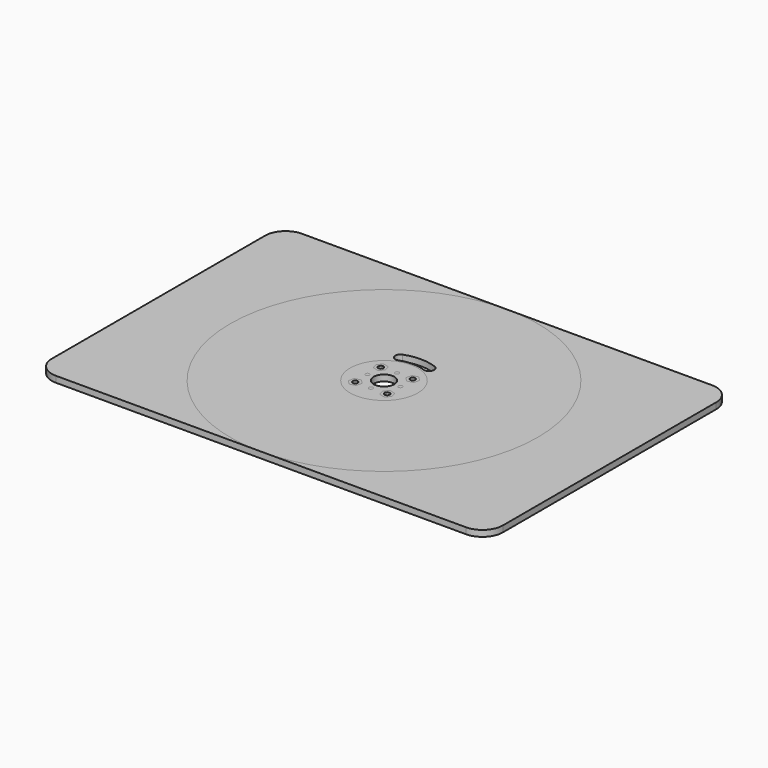
from build123d import *

# Parameters (mm, degrees)
F12_DEPTH = 3
F2_W      = 29
F2_H      = 59.5
F2_R      = 1.25
F6_R      = 2
F13_DEPTH = 25
F3_R      = 75
F14_DEPTH = 3
F5_R      = 2
F7_R      = 30
F15_DEPTH = 25
F16_DEPTH = 3
F0_R      = 5
F0_R_2    = 1.25
F17_DEPTH = 25
F9_R      = 16.5
F18_DEPTH = 3
F11_R     = 1
F19_DEPTH = 25
F20_DEPTH = 3
F10_R     = 2
F21_DEPTH = 25
F22_DEPTH = 3
F1_R      = 5
F23_DEPTH = 25


with BuildPart() as f12:
    # F4 (on Top) → F12 (new body)
    with BuildSketch(Plane.XY):
        with BuildLine():
            Line((100, 75), (-100, 75))
            ThreePointArc((-100, 75), (-107.0710678119, 72.0710678119), (-110, 65))
            Line((-110, 65), (-110, -65))
            ThreePointArc((-110, -65), (-107.0710678119, -72.0710678119), (-100, -75))
            Line((-100, -75), (100, -75))
            ThreePointArc((100, -75), (107.0710678119, -72.0710678119), (110, -65))
            Line((110, -65), (110, 65))
            ThreePointArc((110, 65), (107.0710678119, 72.0710678119), (100, 75))
        make_face()
    extrude(amount=F12_DEPTH)

    # F2 (on Top) + F6 (on Top) + F8 (on Top) → F13 (cut)
    with BuildSketch(Plane.XY):
        with Locations((0, -15.25)):
            Rectangle(F2_W, F2_H)
        with Locations((17.3, 4)):
            Circle(F2_R)
        with Locations((17.3, -18)):
            Circle(F2_R)
        with Locations((17.3, -40)):
            Circle(F2_R)
        with Locations((-17.3, 4)):
            Circle(F2_R)
        with Locations((-17.3, -18)):
            Circle(F2_R)
        with Locations((-17.3, -40)):
            Circle(F2_R)
        with Locations((11, -47.8)):
            Circle(F2_R)
        with Locations((-11, -47.8)):
            Circle(F2_R)
    with BuildSketch(Plane.XY):
        with Locations((38.1837661841, 38.1837661841)):
            Circle(F6_R)
        with Locations((-38.1837661841, 38.1837661841)):
            Circle(F6_R)
        with Locations((-38.1837661841, -38.1837661841)):
            Circle(F6_R)
        with Locations((38.1837661841, -38.1837661841)):
            Circle(F6_R)
    with BuildSketch(Plane.XY):
        with BuildLine():
            ThreePointArc((-7.875, 21.0768682446), (-9.3418742494, 17.8599939952), (-6.125, 16.3931197458))
            ThreePointArc((-6.125, 16.3931197458), (0, 17.5), (6.125, 16.3931197458))
            ThreePointArc((6.125, 16.3931197458), (9.3418742494, 17.8599939952), (7.875, 21.0768682446))
            ThreePointArc((7.875, 21.0768682446), (0, 22.5), (-7.875, 21.0768682446))
        make_face()
    extrude(amount=F13_DEPTH, mode=Mode.SUBTRACT)


with BuildPart() as f14:
    # F3 (on Top) → F14 (new body)
    with BuildSketch(Plane.XY):
        Circle(F3_R)
    extrude(amount=F14_DEPTH)

    # F5 (on Top) + F7 (on Top) → F15 (cut)
    with BuildSketch(Plane.XY):
        with Locations((0, 54)):
            Circle(F5_R)
        with Locations((-54, 0)):
            Circle(F5_R)
        with Locations((0, -54)):
            Circle(F5_R)
        with Locations((54, 0)):
            Circle(F5_R)
    with BuildSketch(Plane.XY):
        Circle(F7_R)
    extrude(amount=F15_DEPTH, mode=Mode.SUBTRACT)


with BuildPart() as f16:
    # F3 (on Top) → F16 (new body)
    with BuildSketch(Plane.XY):
        Circle(F3_R)
    extrude(amount=F16_DEPTH)

    # F0 (on Top) + F8 (on Top) → F17 (cut)
    with BuildSketch(Plane.XY):
        Circle(F0_R)
        with Locations((7.7781745931, 7.7781745931)):
            Circle(F0_R_2)
        with Locations((-7.7781745931, 7.7781745931)):
            Circle(F0_R_2)
        with Locations((-7.7781745931, -7.7781745931)):
            Circle(F0_R_2)
        with Locations((7.7781745931, -7.7781745931)):
            Circle(F0_R_2)
    with BuildSketch(Plane.XY):
        with BuildLine():
            ThreePointArc((-7.875, 21.0768682446), (-9.3418742494, 17.8599939952), (-6.125, 16.3931197458))
            ThreePointArc((-6.125, 16.3931197458), (0, 17.5), (6.125, 16.3931197458))
            ThreePointArc((6.125, 16.3931197458), (9.3418742494, 17.8599939952), (7.875, 21.0768682446))
            ThreePointArc((7.875, 21.0768682446), (0, 22.5), (-7.875, 21.0768682446))
        make_face()
    extrude(amount=F17_DEPTH, mode=Mode.SUBTRACT)


with BuildPart() as f18:
    # F9 (on Top) → F18 (new body)
    with BuildSketch(Plane.XY):
        Circle(F9_R)
    extrude(amount=F18_DEPTH)

    # F0 (on Top) + F11 (on Top) → F19 (cut)
    with BuildSketch(Plane.XY):
        Circle(F0_R)
        with Locations((7.7781745931, 7.7781745931)):
            Circle(F0_R_2)
        with Locations((-7.7781745931, 7.7781745931)):
            Circle(F0_R_2)
        with Locations((-7.7781745931, -7.7781745931)):
            Circle(F0_R_2)
        with Locations((7.7781745931, -7.7781745931)):
            Circle(F0_R_2)
    with BuildSketch(Plane.XY):
        with Locations((0, 8)):
            Circle(F11_R)
        with Locations((-8, 0)):
            Circle(F11_R)
        with Locations((0, -8)):
            Circle(F11_R)
        with Locations((8, 0)):
            Circle(F11_R)
    extrude(amount=F19_DEPTH, mode=Mode.SUBTRACT)


with BuildPart() as f20:
    # F9 (on Top) → F20 (new body)
    with BuildSketch(Plane.XY):
        Circle(F9_R)
    extrude(amount=F20_DEPTH)

    # F0 (on Top) + F10 (on Top) → F21 (cut)
    with BuildSketch(Plane.XY):
        Circle(F0_R)
        with Locations((7.7781745931, 7.7781745931)):
            Circle(F0_R_2)
        with Locations((-7.7781745931, 7.7781745931)):
            Circle(F0_R_2)
        with Locations((-7.7781745931, -7.7781745931)):
            Circle(F0_R_2)
        with Locations((7.7781745931, -7.7781745931)):
            Circle(F0_R_2)
    with BuildSketch(Plane.XY):
        with Locations((0, 8)):
            Circle(F10_R)
        with Locations((-8, 0)):
            Circle(F10_R)
        with Locations((0, -8)):
            Circle(F10_R)
        with Locations((8, 0)):
            Circle(F10_R)
    extrude(amount=F21_DEPTH, mode=Mode.SUBTRACT)


with BuildPart() as f22:
    # F9 (on Top) → F22 (new body)
    with BuildSketch(Plane.XY):
        Circle(F9_R)
    extrude(amount=F22_DEPTH)

    # F11 (on Top) + F1 (on Top) → F23 (cut)
    with BuildSketch(Plane.XY):
        with Locations((0, 8)):
            Circle(F11_R)
        with Locations((-8, 0)):
            Circle(F11_R)
        with Locations((0, -8)):
            Circle(F11_R)
        with Locations((8, 0)):
            Circle(F11_R)
    with BuildSketch(Plane.XY):
        Circle(F1_R)
        Polygon((7.0310283662, 4.9897869139), (9.8194160454, 5.7369331407), (10.5665622722, 8.5253208199), (8.5253208199, 10.5665622722), (5.7369331407, 9.8194160454), (4.9897869139, 7.0310283662), align=None)
        Polygon((-7.0310283662, 4.9897869139), (-4.9897869139, 7.0310283662), (-5.7369331407, 9.8194160454), (-8.5253208199, 10.5665622722), (-10.5665622722, 8.5253208199), (-9.8194160454, 5.7369331407), align=None)
        Polygon((-4.9897869139, -7.0310283662), (-7.0310283662, -4.9897869139), (-9.8194160454, -5.7369331407), (-10.5665622722, -8.5253208199), (-8.5253208199, -10.5665622722), (-5.7369331407, -9.8194160454), align=None)
        Polygon((7.0310283662, -4.9897869139), (4.9897869139, -7.0310283662), (5.7369331407, -9.8194160454), (8.5253208199, -10.5665622722), (10.5665622722, -8.5253208199), (9.8194160454, -5.7369331407), align=None)
    extrude(amount=F23_DEPTH, mode=Mode.SUBTRACT)


solid = Compound([f12.part, f14.part, f16.part, f18.part, f20.part, f22.part])
